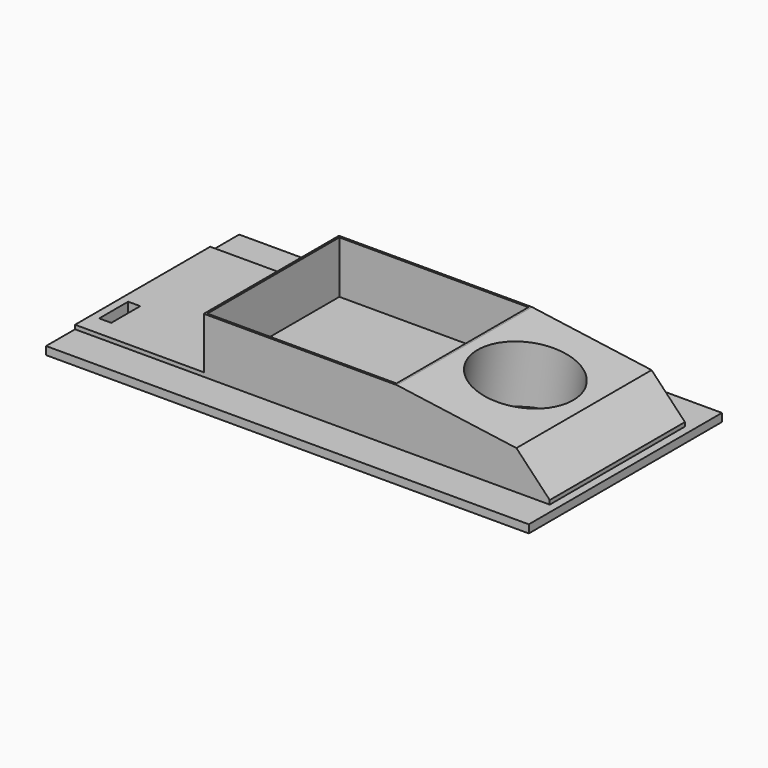
from build123d import *

# Parameters (mm, degrees)
F0_W     = 3048
F0_H     = 1524
F0_W_2   = 76.2
F0_H_2   = 228.6
F1_DEPTH = 50.8
F2_W     = 2997.2
F2_H     = 1066.8
F2_W_2   = 76.2
F2_H_2   = 228.6
F3_DEPTH = 25.4
F5_DEPTH = 1066.8
F6_R     = 304.8
F7_DEPTH = 676.4650551683
F8_W     = 1193.8
F8_H     = 1041.4
F9_DEPTH = 330.2


with BuildPart() as f1:
    # F0 (on Top) → F1 (new body)
    with BuildSketch(Plane.XY):
        with Locations((15.8064851761, -22.5919132233)):
            Rectangle(F0_W, F0_H)
        with Locations((-1419.2935148239, -314.6919132233)):
            Rectangle(F0_W_2, F0_H_2, mode=Mode.SUBTRACT)
    extrude(amount=F1_DEPTH)

    # F2 (on face) → F3 (join)
    with BuildSketch(Plane.XY.offset(50.8)):
        with Locations((-9.5935148239, -22.5919132233)):
            Rectangle(F2_W, F2_H)
        with Locations((-1419.2935148239, -314.6919132233)):
            Rectangle(F2_W_2, F2_H_2, mode=Mode.SUBTRACT)
    extrude(amount=F3_DEPTH)

    # F4 (on face) → F5 (join)
    with BuildSketch(Plane(origin=(0, 510.8080867767, 0), x_dir=(-1, 0, 0), z_dir=(0, 1, 0))):
        Polygon((-1278.5927280739, 296.7200463045), (-1489.0064851761, 76.2), (695.3935148239, 76.2), (695.3935148239, 401.3227591385), (-523.8064851761, 401.3227591385), align=None)
    extrude(amount=-F5_DEPTH)

    # F6 (on face) → F7 (cut, through all)
    with BuildSketch(Plane(origin=(64.4402743808, 0, 464.9844279694), x_dir=(0.9905331272, 0, -0.1372739014), z_dir=(0.1372739014, 0, 0.9905331272))):
        with Locations((833.8910219943, 0)):
            Circle(F6_R)
    extrude(amount=-F7_DEPTH, mode=Mode.SUBTRACT)

    # F8 (on face) → F9 (cut)
    with BuildSketch(Plane.XY.offset(401.3227591385)):
        with Locations((-85.7935148239, -22.5919132233)):
            Rectangle(F8_W, F8_H)
    extrude(amount=-F9_DEPTH, mode=Mode.SUBTRACT)


solid = f1.part
